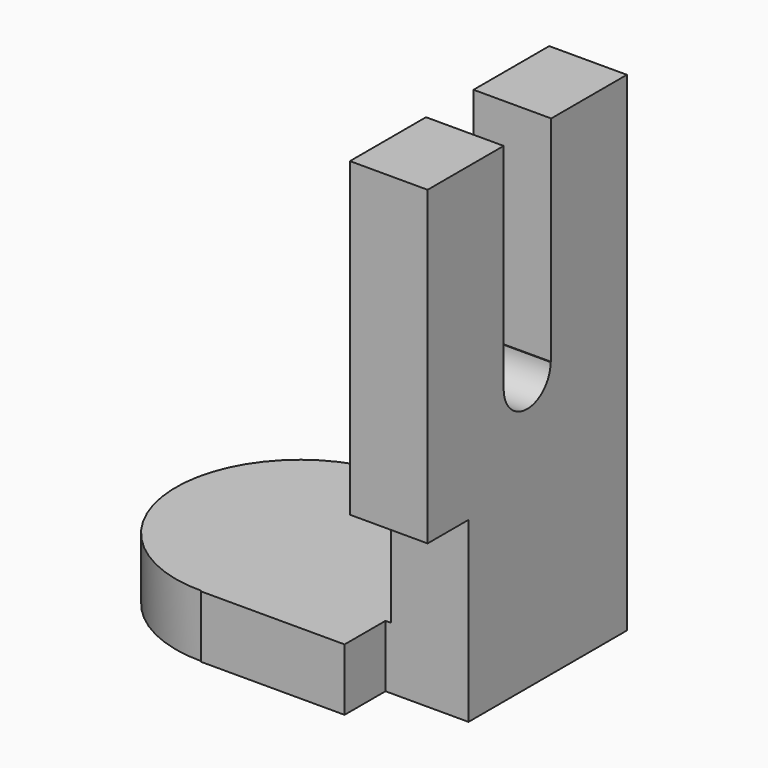
from build123d import *

# Parameters (mm, degrees)
F1_DEPTH = 76.2
F3_DEPTH = 107.7030838857
F5_W     = 15.6415318966
F5_H     = 54.425964132
F6_DEPTH = 25.4
F8_DEPTH = 149.6723981032


# Not quite as in the source:
# - a feature of the source that left no trace in its solid (it failed there, or was rolled back) is left out


with BuildPart() as f1:
    # F0 (on Front) → F1 (new body)
    with BuildSketch(Plane.XZ):
        Polygon((55.1925264299, 74.4524151087), (31.4290784299, 74.4524151087), (31.4290784299, -56.2465488911), (-52.5095574558, -56.2465488911), (-52.5095574558, -75.2189829946), (55.1925264299, -75.2189829946), align=None)
    extrude(amount=F1_DEPTH)

    # F2 (on face) → F3 (cut, through all)
    with BuildSketch(Plane.YZ.offset(55.1925264299)):
        with BuildLine():
            Line((-47.1170713552, 8.9112932328), (-29.1559303752, 8.9112932328))
            ThreePointArc((-29.1559303752, 8.9112932328), (-38.1365008652, 17.8918637228), (-47.1170713552, 8.9112932328))
        make_face()
        with BuildLine():
            ThreePointArc((-47.1170713552, 8.9112932328), (-38.1365008652, -0.0692772572), (-29.1559303752, 8.9112932328))
            Line((-29.1559303752, 8.9112932328), (-47.1170713552, 8.9112932328))
        make_face()
        with BuildLine():
            ThreePointArc((-47.1170713552, 8.9112932328), (-38.1365008652, 17.8918637228), (-29.1559303752, 8.9112932328))
            Line((-29.1559303752, 8.9112932328), (-28.9377495646, 8.9112932328))
            Line((-28.9377495646, 8.9112932328), (-28.9377495646, 74.4524151087))
            Line((-28.9377495646, 74.4524151087), (-47.1170713552, 74.4524151087))
            Line((-47.1170713552, 74.4524151087), (-47.1170713552, 8.9112932328))
        make_face()
    extrude(amount=-F3_DEPTH, mode=Mode.SUBTRACT)

    # F5 (on face) → F6 (cut)
    with BuildSketch(Plane.YZ.offset(55.1925264299)):
        with Locations((-68.3792340517, -48.0060009286)):
            Rectangle(F5_W, F5_H)
    extrude(amount=-F6_DEPTH, mode=Mode.SUBTRACT)

    # F7 (on face) → F8 (cut, through all)
    with BuildSketch(Plane(origin=(0, 0, -75.2189829946), x_dir=(1, 0, 0), z_dir=(0, 0, -1))):
        with BuildLine():
            ThreePointArc((-17.3657385867, 0), (-52.4302228968, 39.5091264656), (-14.1626540173, 75.9245394945))
            Line((-14.1626540173, 75.9245394945), (-14.1626540173, 76.2))
            Line((-14.1626540173, 76.2), (-52.5095574558, 76.2))
            Line((-52.5095574558, 76.2), (-52.5095574558, 0))
            Line((-52.5095574558, 0), (-17.3657385867, 0))
        make_face()
    extrude(amount=-F8_DEPTH, mode=Mode.SUBTRACT)


solid = f1.part
